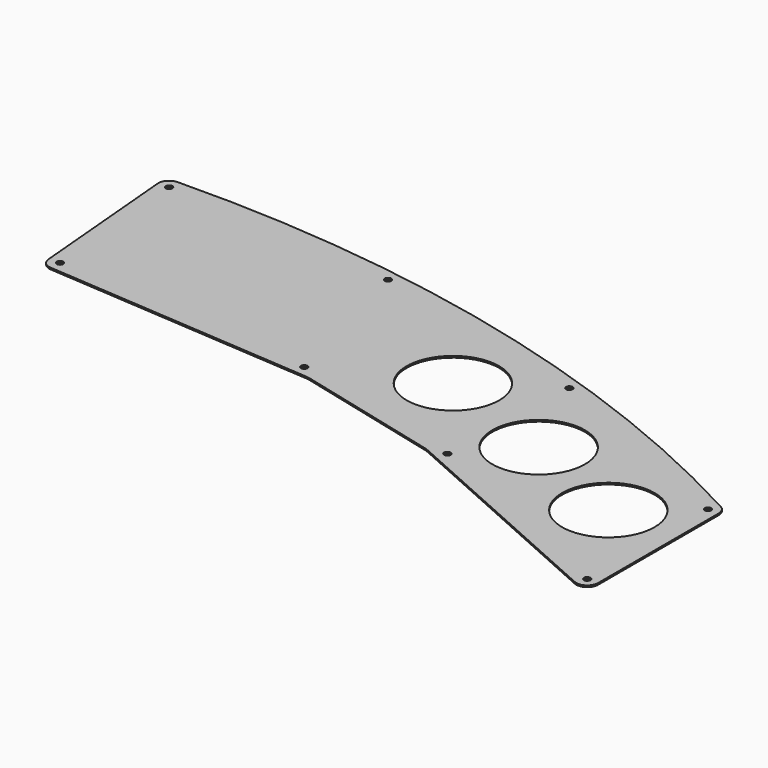
from build123d import *

# Parameters (mm, degrees)
F1_DEPTH = 1.5
F2_R     = 42.5
F3_DEPTH = 1.501
F4_R     = 10
F5_R     = 20
F7_D     = 6


with BuildPart() as f1:
    # F0 (on Top) → F1 (new body)
    with BuildSketch(Plane.XY):
        with BuildLine():
            Line((0, 36.5856099731), (0, 196.5856099731))
            ThreePointArc((0, 196.5856099731), (-307.3351576975, 315.2560594706), (-635, 349.5099039223))
            Line((-635, 349.5099039223), (-621.0269461922, 189.7971680702))
            Line((-621.0269461922, 189.7971680702), (-361.6779078132, 171.4103170113))
            Line((-361.6779078132, 171.4103170113), (-225.8692382849, 137.4102393502))
            Line((-225.8692382849, 137.4102393502), (0, 36.5856099731))
        make_face()
    extrude(amount=F1_DEPTH)

    # F2 (on face) → F3 (cut, through all)
    with BuildSketch(Plane.XY.offset(1.5)):
        with Locations((-275.0559937421, 229.17509395)):
            Circle(F2_R)
        with Locations((-165, 190)):
            Circle(F2_R)
        with Locations((-65, 145)):
            Circle(F2_R)
    extrude(amount=-F3_DEPTH, mode=Mode.SUBTRACT)

    # F4
    f4_edges = [f1.edges().sort_by_distance(p)[0] for p in [
        (0, 196.58561, 0.75),
        (-635, 349.509904, 0.75),
        (-621.026946, 189.797168, 0.75),
        (0, 36.58561, 0.75),
    ]]
    fillet(f4_edges, radius=F4_R)

    # F5
    f5_edges = [f1.edges().sort_by_distance(p)[0] for p in [
        (-361.677908, 171.410317, 0.75),
        (-225.869238, 137.410239, 0.75),
    ]]
    fillet(f5_edges, radius=F5_R)

    # F7 (through all)
    with Locations(Plane.XY.offset(1.5)):
        with Locations((-624.1092854766, 339.7655997622), (-611.8086529213, 199.1687262985), (-411.8395238612, 325.6409079413), (-374.0631195885, 182.3134808013), (-205.1081070963, 275.4405101573), (-209.8076952351, 141.1916790514), (-10, 190.6420127613), (-10, 52.0005303507)):
            Hole(F7_D / 2)


solid = f1.part
